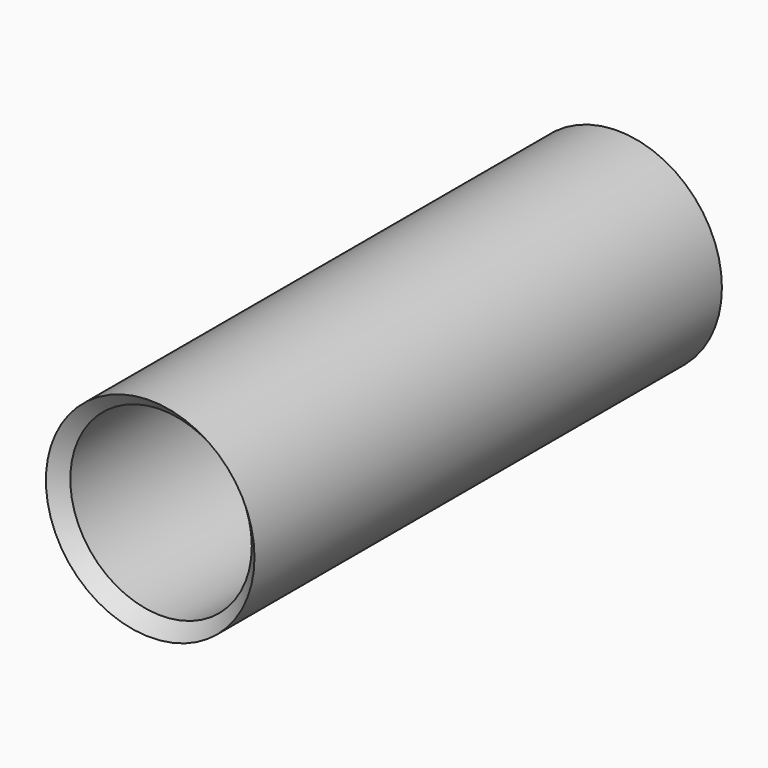
from build123d import *

# Parameters (mm, degrees)
F0_R     = 19.5456573821
F1_DEPTH = 112.014
F2_T     = -2.54


# Not quite as in the source:
# - a fillet or chamfer that OpenCascade refuses, or shapes differently, is made with other operations: its cross-section is extruded or revolved along the edge and cut away or added


with BuildPart() as f1:
    # F0 (on Front) → F1 (new body)
    with BuildSketch(Plane.XZ):
        Circle(F0_R)
    extrude(amount=F1_DEPTH)

    # F2
    f2_openings = [f1.faces().sort_by_distance(p)[0] for p in [
        (0, -112.014, 0),
    ]]
    offset(amount=F2_T, openings=f2_openings)

    # F3: chamfer of 5.08 on 1 edges, made by hand

    # F3_s1 → F3_t2 (revolve, cut)
    with BuildSketch(Plane.XY):
        Polygon((22.0856573821, -112.014), (17.0056573821, -106.934), (17.0056573821, -112.014), align=None)
    revolve(axis=Axis((0, -112.014, 0), (0, -1, 0)), mode=Mode.SUBTRACT)


solid = f1.part
